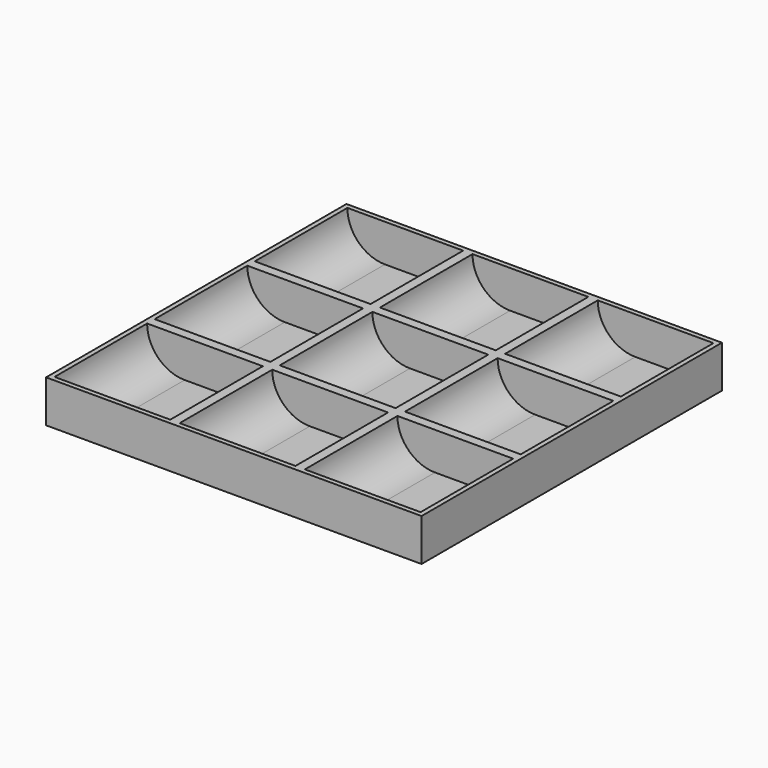
from build123d import *

# Parameters (mm, degrees)
F0_W     = 24.66
F0_H     = 24.66
F0_W_2   = 24.68
F0_H_2   = 24.68
F1_DEPTH = 8
F2_DEPTH = 1
F3_R     = 7.99999


# Not quite as in the source:
# - a fillet or chamfer is up to 0.001 mm smaller than in the source, because OpenCascade refuses the exact size


with BuildPart() as f1:
    # F0 (on Top) → F1 (new body)
    with BuildSketch(Plane.XY):
        Polygon((-40, -40), (40, -40), (40, 40), (-40, 40), (-40, -13.34), align=None)
        with Locations((-26.67, -26.67)):
            Rectangle(F0_W, F0_H, mode=Mode.SUBTRACT)
        with Locations((0, -26.67)):
            Rectangle(F0_W_2, F0_H, mode=Mode.SUBTRACT)
        with Locations((26.67, -26.67)):
            Rectangle(F0_W, F0_H, mode=Mode.SUBTRACT)
        with Locations((-26.67, 0)):
            Rectangle(F0_W, F0_H_2, mode=Mode.SUBTRACT)
        with Locations((-26.67, 26.67)):
            Rectangle(F0_W, F0_H, mode=Mode.SUBTRACT)
        Rectangle(F0_W_2, F0_H_2, mode=Mode.SUBTRACT)
        with Locations((26.67, 0)):
            Rectangle(F0_W, F0_H_2, mode=Mode.SUBTRACT)
        with Locations((0, 26.67)):
            Rectangle(F0_W_2, F0_H, mode=Mode.SUBTRACT)
        with Locations((26.67, 26.67)):
            Rectangle(F0_W, F0_H, mode=Mode.SUBTRACT)
    extrude(amount=F1_DEPTH)

    # F0 (on Top) → F2 (join)
    with BuildSketch(Plane.XY):
        Polygon((-40, -40), (40, -40), (40, 40), (-40, 40), (-40, -13.34), align=None)
        with Locations((-26.67, -26.67)):
            Rectangle(F0_W, F0_H, mode=Mode.SUBTRACT)
        with Locations((0, -26.67)):
            Rectangle(F0_W_2, F0_H, mode=Mode.SUBTRACT)
        with Locations((26.67, -26.67)):
            Rectangle(F0_W, F0_H, mode=Mode.SUBTRACT)
        with Locations((-26.67, 0)):
            Rectangle(F0_W, F0_H_2, mode=Mode.SUBTRACT)
        with Locations((-26.67, 26.67)):
            Rectangle(F0_W, F0_H, mode=Mode.SUBTRACT)
        Rectangle(F0_W_2, F0_H_2, mode=Mode.SUBTRACT)
        with Locations((26.67, 0)):
            Rectangle(F0_W, F0_H_2, mode=Mode.SUBTRACT)
        with Locations((0, 26.67)):
            Rectangle(F0_W_2, F0_H, mode=Mode.SUBTRACT)
        with Locations((26.67, 26.67)):
            Rectangle(F0_W, F0_H, mode=Mode.SUBTRACT)
        Rectangle(F0_W_2, F0_H_2)
        with Locations((-26.67, 0)):
            Rectangle(F0_W, F0_H_2)
        with Locations((0, -26.67)):
            Rectangle(F0_W_2, F0_H)
        with Locations((26.67, 0)):
            Rectangle(F0_W, F0_H_2)
        with Locations((0, 26.67)):
            Rectangle(F0_W_2, F0_H)
        with Locations((-26.67, -26.67)):
            Rectangle(F0_W, F0_H)
        with Locations((-26.67, 26.67)):
            Rectangle(F0_W, F0_H)
        with Locations((26.67, -26.67)):
            Rectangle(F0_W, F0_H)
        with Locations((26.67, 26.67)):
            Rectangle(F0_W, F0_H)
    extrude(amount=-F2_DEPTH)

    # F3 (radius 8 in the source; OpenCascade refuses exactly that, so slightly less here)
    f3_edges = [f1.edges().sort_by_distance(p)[0] for p in [
        (14.34, -26.67, 0),
        (14.34, 0, 0),
        (14.34, 26.67, 0),
        (-12.34, 26.67, 0),
        (-12.34, 0, 0),
        (-12.34, -26.67, 0),
        (-39, -26.67, 0),
        (-39, 0, 0),
        (-39, 26.67, 0),
        (12.34, -26.67, 0),
        (12.34, 0, 0),
        (12.34, 26.67, 0),
        (-14.34, 26.67, 0),
        (-14.34, 0, 0),
        (-14.34, -26.67, 0),
        (39, 26.67, 0),
        (39, 0, 0),
        (39, -26.67, 0),
    ]]
    fillet(f3_edges, radius=F3_R)


solid = f1.part
